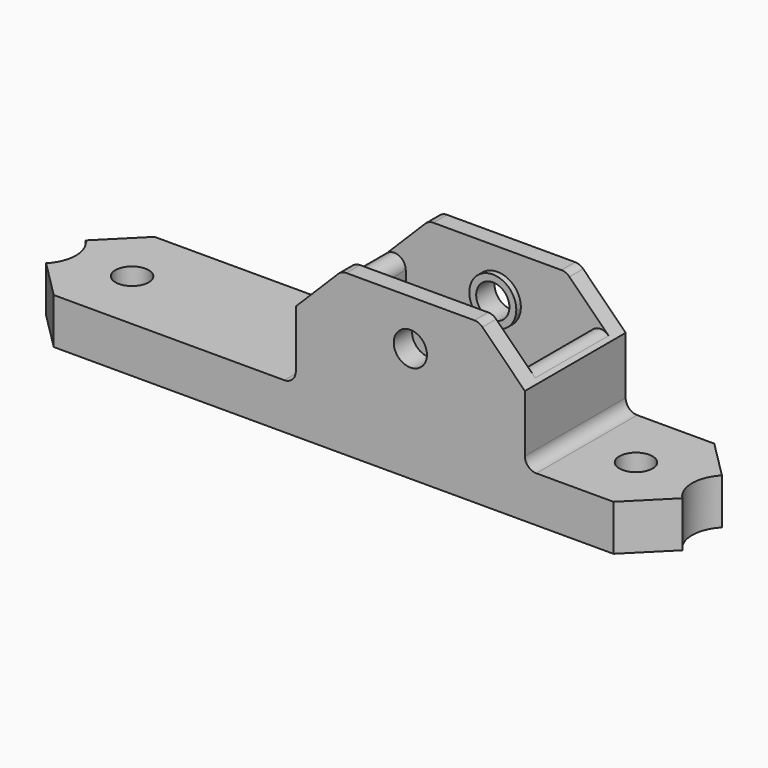
from build123d import *

# Parameters (mm, degrees)
F0_R        = 1.45
F0_W        = 20
F0_H        = 11
F0_W_2      = 16
F0_H_2      = 8
F1_DEPTH    = 4
F2_DEPTH    = 10
F3_R        = 1.45
F4_DEPTH    = 25
F3_R_2      = 2.05
F5_DEPTH    = 11
F0_W_3      = 5
F0_H_3      = 7
F6_DEPTH    = 25
F7_T1_DEPTH = 31.5734639037
F7_T3_DEPTH = 24.5734639037
F8_R        = 1


# Not quite as in the source:
# - a fillet or chamfer that OpenCascade refuses, or shapes differently, is made with other operations: its cross-section is extruded or revolved along the edge and cut away or added


with BuildPart() as f1:
    # F0 (on Top) → F1 (new body)
    with BuildSketch(Plane.XY):
        with BuildLine():
            ThreePointArc((-28.4361224622, 2.6766185844), (-27.3113181327, 1.54304563), (-26.9, 0))
            ThreePointArc((-26.9, 0), (-27.3113181327, -1.54304563), (-28.4361224622, -2.6766185844))
            Line((-28.4361224622, -2.6766185844), (-28.4361224622, -5.5))
            Line((-28.4361224622, -5.5), (-3.3, -5.5))
            Line((-3.3, -5.5), (-3.3, 5.5))
            Line((-3.3, 5.5), (-28.4361224622, 5.5))
            Line((-28.4361224622, 5.5), (-28.4361224622, 2.6766185844))
        make_face()
        with Locations((-22, 0)):
            Circle(F0_R, mode=Mode.SUBTRACT)
        with BuildLine():
            Line((28.4361224622, 5.5), (16.7, 5.5))
            Line((16.7, 5.5), (16.7, -5.5))
            Line((16.7, -5.5), (28.4361224622, -5.5))
            Line((28.4361224622, -5.5), (28.4361224622, -2.6766185844))
            ThreePointArc((28.4361224622, -2.6766185844), (26.9, 0), (28.4361224622, 2.6766185844))
            Line((28.4361224622, 2.6766185844), (28.4361224622, 5.5))
        make_face()
        with Locations((22, 0)):
            Circle(F0_R, mode=Mode.SUBTRACT)
        with Locations((6.7, 0)):
            Rectangle(F0_W, F0_H)
        with Locations((6.7, 0)):
            Rectangle(F0_W_2, F0_H_2, mode=Mode.SUBTRACT)
    extrude(amount=-F1_DEPTH)

    # F0 (on Top) → F2 (join)
    with BuildSketch(Plane.XY):
        with Locations((6.7, 0)):
            Rectangle(F0_W, F0_H)
        with Locations((6.7, 0)):
            Rectangle(F0_W_2, F0_H_2, mode=Mode.SUBTRACT)
    extrude(amount=F2_DEPTH)

    # F3 (on face) → F4 (cut)
    with BuildSketch(Plane.XZ.offset(5.5)):
        with Locations((6.7, 6)):
            Circle(F3_R)
    extrude(amount=-F4_DEPTH, mode=Mode.SUBTRACT)

    # F3 (on face) → F5 (join, through all)
    with BuildSketch(Plane.XZ.offset(5.5)):
        with Locations((6.7, 6)):
            Circle(F3_R_2)
        with Locations((6.7, 6)):
            Circle(F3_R, mode=Mode.SUBTRACT)
    extrude(amount=-F5_DEPTH)

    # F0 (on Top) → F6 (cut)
    with BuildSketch(Plane.XY):
        with Locations((6.7, 0)):
            Rectangle(F0_W_3, F0_H_3)
    extrude(amount=F6_DEPTH, mode=Mode.SUBTRACT)

    # F7: chamfer of 4 on 6 edges, made by hand

    # F7_s2 → F7_t1 (cut)
    with BuildSketch(Plane.XZ.offset(-15.7867319519)):
        Polygon((-3.3, 6), (0.7, 10), (-3.3, 10), align=None)
        Polygon((12.7, 10), (16.7, 6), (16.7, 10), align=None)
    extrude(amount=F7_T1_DEPTH, mode=Mode.SUBTRACT)

    # F7_s4 → F7_t3 (cut)
    with BuildSketch(Plane.XY.offset(-14.2867319519)):
        Polygon((-28.4361224622, -1.5), (-24.4361224622, -5.5), (-28.4361224622, -5.5), align=None)
        Polygon((-28.4361224622, 1.5), (-24.4361224622, 5.5), (-28.4361224622, 5.5), align=None)
        Polygon((24.4361224622, -5.5), (28.4361224622, -1.5), (28.4361224622, -5.5), align=None)
        Polygon((24.4361224622, 5.5), (28.4361224622, 1.5), (28.4361224622, 5.5), align=None)
    extrude(amount=F7_T3_DEPTH, mode=Mode.SUBTRACT)

    # F8
    f8_edges = [f1.edges().sort_by_distance(p)[0] for p in [
        (-1.3, 0, 8),
        (14.7, 0, 8),
        (0.7, 4.75, 10),
        (0.7, -4.75, 10),
        (12.7, -4.75, 10),
        (12.7, 4.75, 10),
        (-3.3, 0, 0),
        (16.7, 0, 0),
    ]]
    fillet(f8_edges, radius=F8_R)


solid = f1.part
